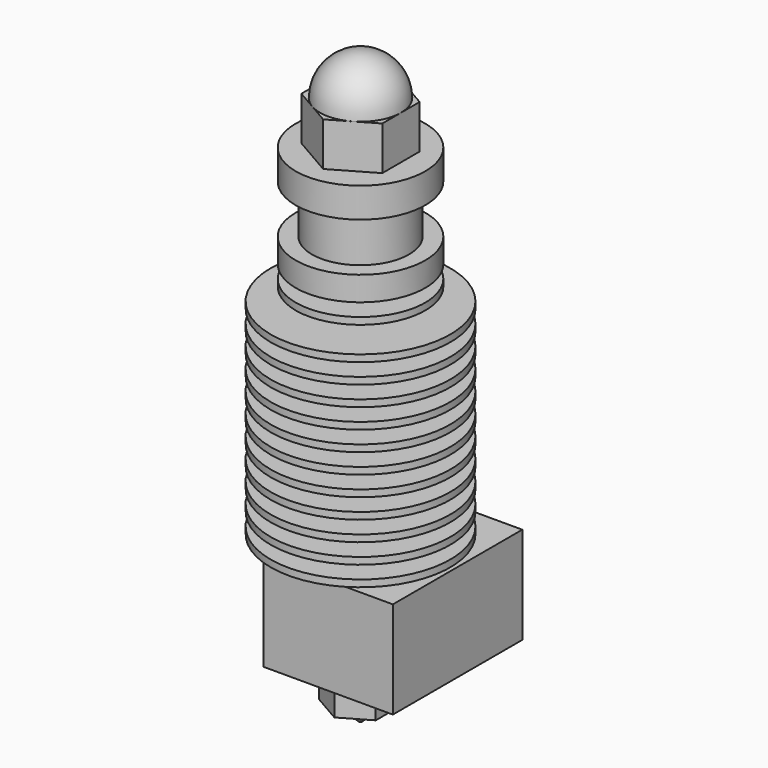
from build123d import *

# Parameters (mm, degrees)
F0_W          = 2.5
F0_H          = 3
F3_START      = 41.25
F2_R          = 4
F3_DEPTH      = 5.4
F0_W_2        = 8
F0_H_2        = 12
F4_DEPTH      = 5
F4_DEPTH_BACK = 15
F6_START      = -15.85
F5_R          = 2.25
F6_DEPTH      = 3.3
F8_R          = 2.25
F9_DEPTH      = 2
F9_TAPER      = 45


with BuildPart() as f1:
    # F0 (on Front) → F1 (revolve)
    with BuildSketch(Plane.XZ):
        Polygon((-6, 37.55), (0, 37.55), (0, 41.25), (-8, 41.25), (-8, 37.55), align=None)
        Polygon((-0.4310491562, 31.55), (0, 31.55), (0, 37.55), (-6, 37.55), (-6, 31.55), align=None)
        with BuildLine():
            Line((-3.5, 28.55), (0, 28.55))
            Line((0, 28.55), (0, 31.4520410289))
            ThreePointArc((0, 31.4520410289), (-0.2160659165, 31.4986384615), (-0.4310491562, 31.55))
            Line((-0.4310491562, 31.55), (-6, 31.55))
            Line((-6, 31.55), (-8, 31.55))
            Line((-8, 31.55), (-8, 28.55))
            Line((-8, 28.55), (-3.5, 28.55))
        make_face()
        Polygon((-3.6961471103, 26.95), (0, 26.95), (0, 28.55), (-3.5, 28.55), align=None)
        Polygon((-5.3021015762, 13.85), (0, 13.85), (0, 14.7), (-5.1978984238, 14.7), align=None)
        Polygon((0, -0.85), (0, 0), (-7, 0), (-11.1, 0), (-11.1, -0.85), (-2.5, -0.85), align=None)
        Polygon((-6.8038528897, 1.6), (0, 1.6), (0, 2.45), (-6.6996497373, 2.45), align=None)
        Polygon((-4.5971978984, 19.6), (0, 19.6), (0, 21.2), (-4.4010507881, 21.2), align=None)
        Polygon((-3.8003502627, 26.1), (0, 26.1), (0, 26.95), (-3.6961471103, 26.95), align=None)
        Polygon((-5.9028021016, 8.95), (0, 8.95), (0, 9.8), (-5.7985989492, 9.8), align=None)
        Polygon((-6.503502627, 4.05), (0, 4.05), (0, 4.9), (-6.3992994746, 4.9), align=None)
        Polygon((-3.996497373, 24.5), (0, 24.5), (0, 26.1), (-3.8003502627, 26.1), align=None)
        Polygon((-5.7985989492, 9.8), (0, 9.8), (0, 11.4), (-5.6024518389, 11.4), align=None)
        Polygon((-5.0017513135, 16.3), (0, 16.3), (0, 17.15), (-4.8975481611, 17.15), align=None)
        Polygon((-4.1007005254, 23.65), (0, 23.65), (0, 24.5), (-3.996497373, 24.5), align=None)
        Polygon((-6.2031523643, 6.5), (0, 6.5), (0, 7.35), (-6.0989492119, 7.35), align=None)
        Polygon((-6.0989492119, 7.35), (0, 7.35), (0, 8.95), (-5.9028021016, 8.95), align=None)
        Polygon((-6.6996497373, 2.45), (0, 2.45), (0, 4.05), (-6.503502627, 4.05), align=None)
        Polygon((-7, 0), (0, 0), (0, 1.6), (-6.8038528897, 1.6), align=None)
        Polygon((-6.3992994746, 4.9), (0, 4.9), (0, 6.5), (-6.2031523643, 6.5), align=None)
        Polygon((-4.8975481611, 17.15), (0, 17.15), (0, 18.75), (-4.7014010508, 18.75), align=None)
        Polygon((-4.2968476357, 22.05), (0, 22.05), (0, 23.65), (-4.1007005254, 23.65), align=None)
        Polygon((-5.4982486865, 12.25), (0, 12.25), (0, 13.85), (-5.3021015762, 13.85), align=None)
        Polygon((-4.7014010508, 18.75), (0, 18.75), (0, 19.6), (-4.5971978984, 19.6), align=None)
        Polygon((-4.4010507881, 21.2), (0, 21.2), (0, 22.05), (-4.2968476357, 22.05), align=None)
        Polygon((-5.1978984238, 14.7), (0, 14.7), (0, 16.3), (-5.0017513135, 16.3), align=None)
        Polygon((-5.6024518389, 11.4), (0, 11.4), (0, 12.25), (-5.4982486865, 12.25), align=None)
        Polygon((-8, 26.1), (-3.8003502627, 26.1), (-3.6961471103, 26.95), (-8, 26.95), align=None)
        Polygon((-11.1, 23.65), (-4.1007005254, 23.65), (-3.996497373, 24.5), (-11.1, 24.5), align=None)
        Polygon((-11.1, 21.2), (-4.4010507881, 21.2), (-4.2968476357, 22.05), (-11.1, 22.05), align=None)
        Polygon((-11.1, 18.75), (-4.7014010508, 18.75), (-4.5971978984, 19.6), (-11.1, 19.6), align=None)
        Polygon((-11.1, 16.3), (-5.0017513135, 16.3), (-4.8975481611, 17.15), (-11.1, 17.15), align=None)
        Polygon((-11.1, 13.85), (-5.3021015762, 13.85), (-5.1978984238, 14.7), (-11.1, 14.7), align=None)
        Polygon((-11.1, 11.4), (-5.6024518389, 11.4), (-5.4982486865, 12.25), (-11.1, 12.25), align=None)
        Polygon((-11.1, 8.95), (-5.9028021016, 8.95), (-5.7985989492, 9.8), (-11.1, 9.8), align=None)
        Polygon((-11.1, 6.5), (-6.2031523643, 6.5), (-6.0989492119, 7.35), (-11.1, 7.35), align=None)
        Polygon((-11.1, 4.05), (-6.503502627, 4.05), (-6.3992994746, 4.9), (-11.1, 4.9), align=None)
        Polygon((-11.1, 1.6), (-6.8038528897, 1.6), (-6.6996497373, 2.45), (-11.1, 2.45), align=None)
        with Locations((-1.25, -2.35)):
            Rectangle(F0_W, F0_H)
    revolve(axis=Axis((0, 0, 34.55), (0, 0, 1)))


with BuildPart() as f1b:
    # F0 (on Front) → F1, piece 2 (revolve)
    with BuildSketch(Plane.XZ):
        with BuildLine():
            Line((0, 46.65), (0, 51.65))
            ThreePointArc((0, 51.65), (-3.5355339059, 50.1855339059), (-5, 46.65))
            Line((-5, 46.65), (0, 46.65))
        make_face()
    revolve(axis=Axis((0, 0, 34.55), (0, 0, 1)))

    # F2 (on Top) → F3 (join)
    with BuildSketch(Plane.XY.offset(F3_START)):
        Polygon((5, -2.8867513459), (5, 2.8867513459), (0, 5.7735026919), (-5, 2.8867513459), (-5, -2.8867513459), (0, -5.7735026919), align=None)
        Circle(F2_R, mode=Mode.SUBTRACT)
        Circle(F2_R)
    extrude(amount=F3_DEPTH)


with BuildPart() as f4:
    # F0 (on Front) → F4 (new body, two sides)
    with BuildSketch(Plane.XZ) as f4_sk:
        Polygon((0, -15.85), (0, -3.85), (-2.5, -3.85), (-8, -3.85), (-8, -15.85), align=None)
        with Locations((4, -9.85)):
            Rectangle(F0_W_2, F0_H_2)
    extrude(amount=F4_DEPTH)
    extrude(f4_sk.sketch, amount=-F4_DEPTH_BACK)


with BuildPart() as f6:
    # F5 (on Top) → F6 (new body)
    with BuildSketch(Plane.XY.offset(F6_START)):
        Polygon((3.5, -2.0207259422), (3.5, 2.0207259422), (0, 4.0414518843), (-3.5, 2.0207259422), (-3.5, -2.0207259422), (0, -4.0414518843), align=None)
        Circle(F5_R, mode=Mode.SUBTRACT)
        Circle(F5_R)
    extrude(amount=-F6_DEPTH)

    # F8 (on offset) → F9 (join)
    with BuildSketch(Plane(origin=(0, 0, -19.15), x_dir=(1, 0, 0), z_dir=(0, 0, -1))):
        Circle(F8_R)
    extrude(amount=F9_DEPTH, taper=F9_TAPER)


solid = Compound([f1.part, f1b.part, f4.part, f6.part])
